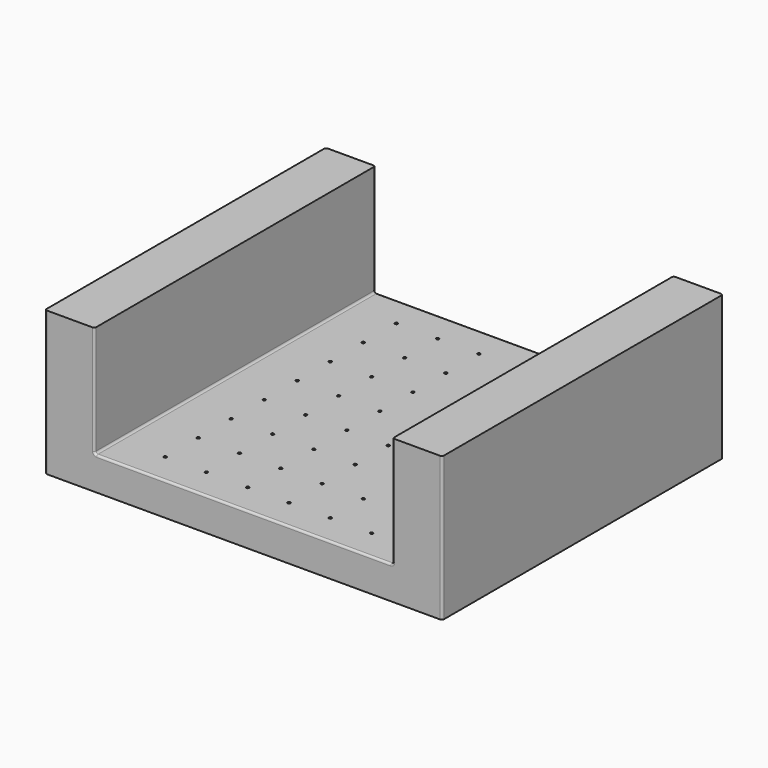
from build123d import *

# Parameters (mm, degrees)
F1_DEPTH = 850
F2_R     = 5
F4_D     = 6.8
F4_DEPTH = 33.75
F4_TIP   = 2.0429261047


with BuildPart() as f1:
    # F0 (on Front) → F1 (new body)
    with BuildSketch(Plane.XZ):
        Polygon((0, 0), (-361, 0), (-361, 269), (-481, 269), (-481, -80), (0, -80), (481, -80), (481, 269), (361, 269), (361, 0), align=None)
    extrude(amount=F1_DEPTH)

    # F2
    f2_edges = [f1.edges().sort_by_distance(p)[0] for p in [
        (-361, -425, 0),
        (361, -425, 0),
        (-361, -850, 134.5),
        (-481, -850, 94.5),
        (481, -850, 94.5),
        (481, 0, 94.5),
        (361, 0, 134.5),
        (-481, 0, 94.5),
        (0, 0, 0),
        (0, -850, 0),
        (361, -850, 134.5),
        (-361, 0, 134.5),
    ]]
    fillet(f2_edges, radius=F2_R)

    # F4
    with Locations(Plane.XY):
        with Locations((50, -675), (50, -775), (-150, -75), (150, -775), (250, -75), (250, -175), (-50, -675), (-150, -675), (-250, -375), (-150, -775), (50, -575), (250, -275), (50, -75), (-150, -475), (-50, -475), (-50, -375), (-250, -275), (150, -75), (-150, -275), (250, -475), (-50, -775), (-250, -75), (250, -375), (-150, -175), (250, -575), (50, -475), (-250, -175), (-250, -575), (-50, -575), (250, -675), (50, -375), (-50, -75), (-50, -275), (-150, -375), (250, -775), (50, -275), (-250, -475), (-250, -775), (150, -175), (50, -175), (-150, -575), (150, -275), (-50, -175), (-250, -675), (150, -375), (150, -475), (150, -675), (150, -575)):
            Hole(F4_D / 2, depth=F4_DEPTH)
            with Locations((0, 0, -(F4_DEPTH + F4_TIP / 2))):  # 118° drill point
                Cone(0, F4_D / 2, F4_TIP, mode=Mode.SUBTRACT)


solid = f1.part
